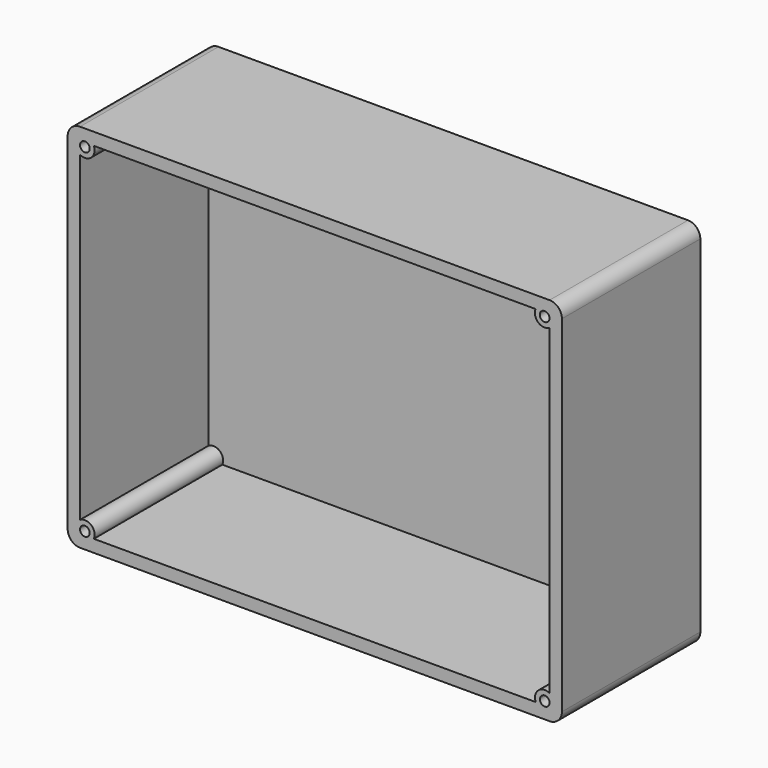
from build123d import *

# Parameters (mm, degrees)
F0_W     = 203.2
F0_H     = 152.4
F1_DEPTH = 71.12
F2_R     = 5.08
F3_T     = 5.08
F4_R     = 4
F5_DEPTH = 71.12
F7_D     = 4
F7_DEPTH = 25.4
F7_TIP   = 1.2017212381


# Not quite as in the source:
# - a shell that OpenCascade refuses in one call is made with other operations: the cavity is built on its own and cut out


with BuildPart() as f1:
    # F0 (on Front) → F1 (new body)
    with BuildSketch(Plane.XZ):
        with Locations((101.6, 76.2)):
            Rectangle(F0_W, F0_H)
    extrude(amount=F1_DEPTH)

    # F2
    f2_edges = [f1.edges().sort_by_distance(p)[0] for p in [
        (0, -35.56, 152.4),
        (0, -35.56, 0),
        (203.2, -35.56, 152.4),
        (203.2, -35.56, 0),
    ]]
    fillet(f2_edges, radius=F2_R)

    # F3: shell of thickness 5.08, made by hand


with BuildPart() as f3_core1:
    # F3_t2: copy of F1
    add(f1.part)

    # the walls: a layer under each face that stays
    f3_faces = [f3_core1.faces().sort_by_distance(p)[0] for p in [
        (0, -35.56, 76.2),
        (101.6, 0, 76.2),
        (101.6, -35.56, 152.4),
        (101.6, -35.56, 0),
        (203.2, -35.56, 76.2),
    ]]
    thicken(f3_faces, amount=-F3_T, mode=Mode.SUBTRACT)


with BuildPart() as f1_1:
    add(f1.part)

    # what is left inside the walls is the cavity
    f3_cavity = [f3_core1.part.solids().sort_by_distance(p)[0] for p in [
        (101.6, -5.1308, 52.493333),
    ]]
    add(f3_cavity, mode=Mode.SUBTRACT)

    # F4 (on Front) → F5 (join)
    with BuildSketch(Plane.XZ):
        with Locations((7.0729700904, 145.7453031343)):
            Circle(F4_R)
        with Locations((196.0783849807, 145.8089049954)):
            Circle(F4_R)
        with Locations((7.0786034794, 6.6475407913)):
            Circle(F4_R)
        with Locations((196.1331322956, 6.6623895618)):
            Circle(F4_R)
    extrude(amount=F5_DEPTH)

    # F7
    with Locations(Plane.XZ.offset(71.12)):
        with Locations((7.0729700904, 145.7453031343), (7.0786034794, 6.6475407913), (196.1331322956, 6.6623895618), (196.0783849807, 145.8089049954)):
            Hole(F7_D / 2, depth=F7_DEPTH)
            with Locations((0, 0, -(F7_DEPTH + F7_TIP / 2))):  # 118° drill point
                Cone(0, F7_D / 2, F7_TIP, mode=Mode.SUBTRACT)


solid = f1_1.part
